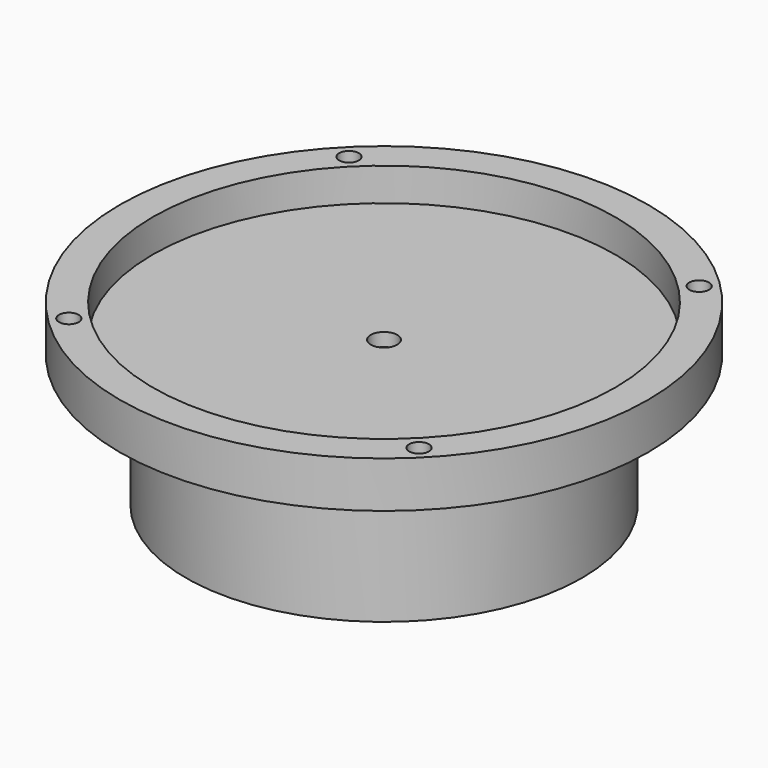
from build123d import *

# Parameters (mm, degrees)
F0_R            = 50.8
F1_DEPTH        = 2.54
F2_R            = 50.8
F2_R_2          = 44.45
F3_DEPTH        = 6.35
F5_D            = 3.7973
F5_COPIES_COUNT = 4
F7_D            = 5.1054
F8_R            = 38.1
F8_R_2          = 2.5527
F9_DEPTH        = 25.4


# Not quite as in the source:
# - a pattern or mirror of a feature is missing from the dataset's text; its kind, count and spacing are read off the source's solid


with BuildPart() as f1:
    # F0 (on Top) → F1 (new body)
    with BuildSketch(Plane.XY):
        Circle(F0_R)
    extrude(amount=F1_DEPTH)

    # F2 (on face) → F3 (join)
    with BuildSketch(Plane.XY.offset(2.54)):
        Circle(F2_R)
        Circle(F2_R_2, mode=Mode.SUBTRACT)
    extrude(amount=F3_DEPTH)

    # F5 (through all)
    with Locations(Plane.XY.offset(8.89)):
        with Locations((-33.675960454, 33.675960454)):
            f5 = Hole(F5_D / 2)

    # F5_copies: F5 ×4 about axis
    f5_copies_axis = Axis((0, 0, 0), (0, 0, 1))
    for i in range(1, F5_COPIES_COUNT):
        add(f5.rotate(f5_copies_axis, i * 360 / F5_COPIES_COUNT), mode=Mode.SUBTRACT)

    # F7 (through all)
    with Locations(Plane.XY.offset(2.54)):
        with Locations((0, 0)):
            Hole(F7_D / 2)

    # F8 (on face) → F9 (join)
    with BuildSketch(Plane(origin=(0, 0, 0), x_dir=(1, 0, 0), z_dir=(0, 0, -1))):
        Circle(F8_R)
        Circle(F8_R_2, mode=Mode.SUBTRACT)
        Circle(F8_R_2)
    extrude(amount=F9_DEPTH)


solid = f1.part
